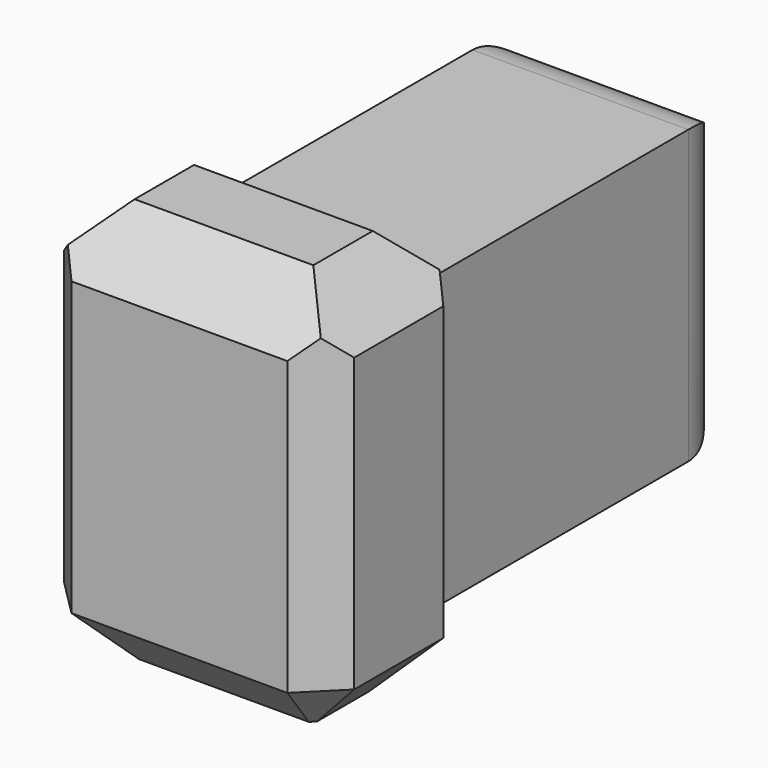
from build123d import *

# Parameters (mm, degrees)
F0_W     = 39.6977961063
F0_H     = 55.2159845829
F1_DEPTH = 25.4
F2_SIZE  = 7.62
F3_SIZE  = 5.08
F4_SIZE  = 7.62
F5_DEPTH = 50.8
F6_R     = 7.62


with BuildPart() as f1:
    # F0 (on Front) → F1 (new body)
    with BuildSketch(Plane.XZ):
        with Locations((19.8488980532, 27.6079922915)):
            Rectangle(F0_W, F0_H)
    extrude(amount=F1_DEPTH)

    # F2
    f2_edges = [f1.edges().sort_by_distance(p)[0] for p in [
        (19.848898, -25.4, 55.215985),
        (0, -12.7, 55.215985),
        (39.697796, -12.7, 55.215985),
        (19.848898, 0, 55.215985),
    ]]
    chamfer(f2_edges, length=F2_SIZE)

    # F3
    f3_edges = [f1.edges().sort_by_distance(p)[0] for p in [
        (39.697796, 0, 23.797992),
        (0, -25.4, 23.797992),
        (39.697796, -25.4, 23.797992),
        (0, 0, 23.797992),
    ]]
    chamfer(f3_edges, length=F3_SIZE)

    # F4
    f4_edges = [f1.edges().sort_by_distance(p)[0] for p in [
        (2.54, -2.54, 0),
        (39.697796, -12.7, 0),
        (0, -12.7, 0),
        (2.54, -22.86, 0),
        (19.848898, -25.4, 0),
        (19.848898, 0, 0),
        (37.157796, -2.54, 0),
        (37.157796, -22.86, 0),
    ]]
    chamfer(f4_edges, length=F4_SIZE)

    # F5 (add): a face of the model
    f5_faces = [f1.faces().sort_by_distance(p)[0] for p in [
        (19.8488980532, 0, 27.6079922915),
    ]]
    extrude(f5_faces, amount=F5_DEPTH)

    # F6
    f6_edges = [f1.edges().sort_by_distance(p)[0] for p in [
        (19.848898, 50.8, 7.62),
        (19.848898, 50.8, 47.595985),
        (5.08, 50.8, 27.607992),
        (34.617796, 50.8, 27.607992),
    ]]
    fillet(f6_edges, radius=F6_R)


solid = f1.part
